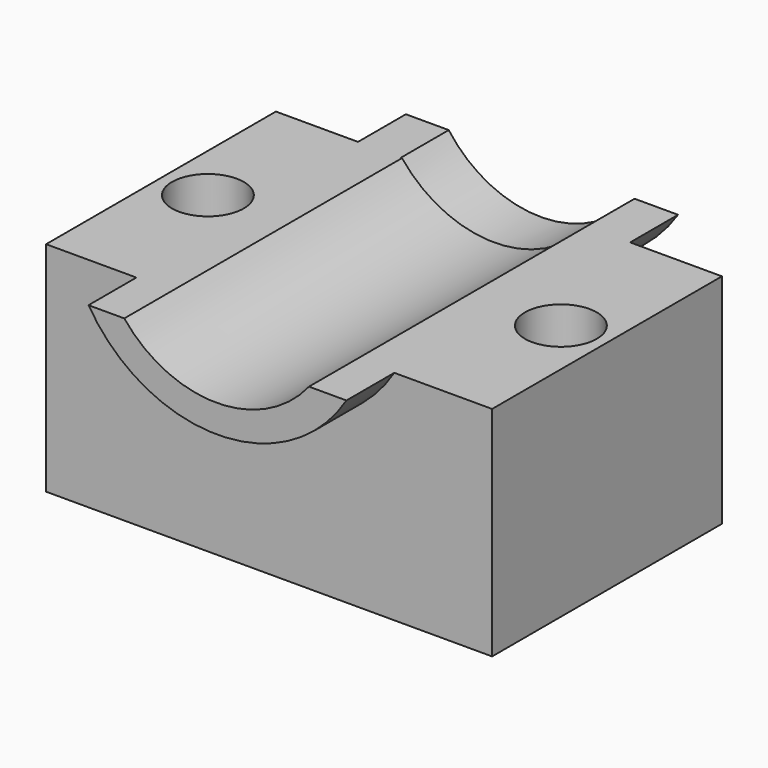
from build123d import *

# Parameters (mm, degrees)
F0_W        = 186.3179504871
F0_H        = 91.0190269351
F1_DEPTH    = 60
F3_DEPTH    = 25
F5_DEPTH    = 25
F7_DEPTH    = 181
F10_D       = 30
F10_ON_F9_D = 30


with BuildPart() as f1:
    # F0 (on Front) → F1 (new body, symmetric)
    with BuildSketch(Plane.XZ):
        with Locations((0.5706548691, -4.2798891664)):
            Rectangle(F0_W, F0_H)
    extrude(amount=F1_DEPTH, both=True)

    # F2 (on face) → F3 (join)
    with BuildSketch(Plane.XZ.offset(60)):
        with BuildLine():
            ThreePointArc((37.2350551188, 41.2296243012), (-1.3436250294, 22.7301151194), (-39.9223051776, 41.2296243012))
            Line((-39.9223051776, 41.2296243012), (-54.8638885904, 41.2296243012))
            ThreePointArc((-54.8638885904, 41.2296243012), (-0.9986385703, 11.1155049194), (52.8666114498, 41.2296243012))
            Line((52.8666114498, 41.2296243012), (37.2350551188, 41.2296243012))
        make_face()
    extrude(amount=F3_DEPTH)

    # F4 (on face) → F5 (join)
    with BuildSketch(Plane(origin=(0, 60, 0), x_dir=(-1, 0, 0), z_dir=(0, 1, 0))):
        with BuildLine():
            Line((-36.6474762559, 41.2296243012), (-55.402355561, 41.2296243012))
            ThreePointArc((-55.402355561, 41.2296243012), (1.44476071, 10.6097235864), (58.291876981, 41.2296243012))
            Line((58.291876981, 41.2296243012), (40.3841994703, 41.2296243012))
            ThreePointArc((40.3841994703, 41.2296243012), (1.8683616072, 21.7640944123), (-36.6474762559, 41.2296243012))
        make_face()
    extrude(amount=F5_DEPTH)

    # F7 (cut): a face of the model
    f7_faces = [f1.faces().sort_by_distance(p)[0] for p in [
        (-1.3436250294, -60, 33.6967312772),
    ]]
    extrude(f7_faces, amount=-F7_DEPTH, mode=Mode.SUBTRACT)

    # F10 (through all)
    with Locations(Plane.XY.offset(41.2296243012)):
        with Locations((-72.9959234595, 0)):
            Hole(F10_D / 2)

    # F10 on F9 (through all)
    with Locations(Plane.XY.offset(41.2296243012)):
        with Locations((74.4606032968, 0)):
            Hole(F10_ON_F9_D / 2)


solid = f1.part
